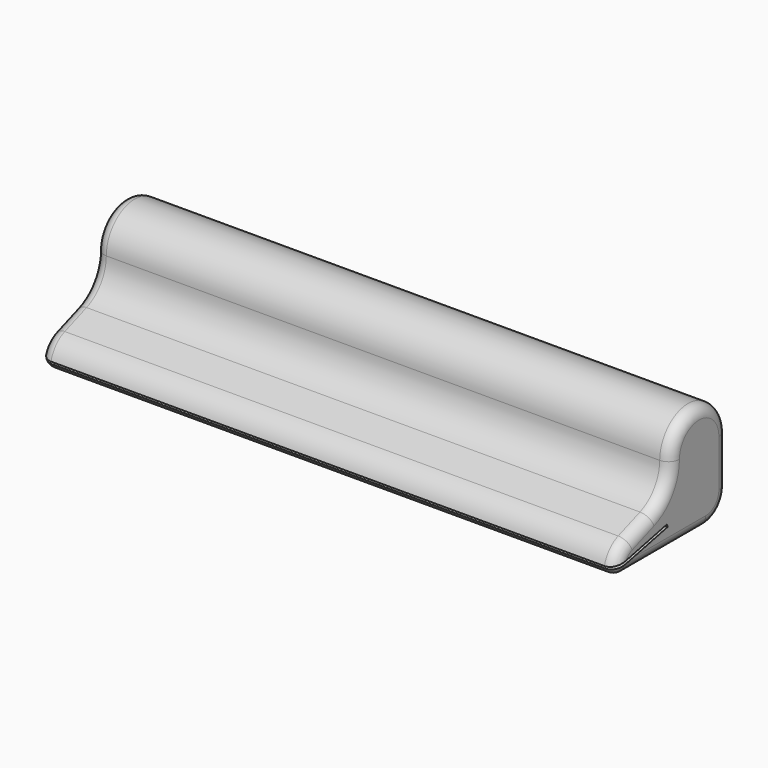
from build123d import *

# Parameters (mm, degrees)
F1_DEPTH     = 105
F2_T1_DEPTH  = 111.9389319908
F3_T1_DEPTH  = 130
F3_T3_DEPTH  = 125.8562768937
F4_T1_DEPTH  = 5.296560543
F4_T3_DEPTH  = 8.5
F4_T5_DEPTH  = 18.6122136018
F4_T8_ANGLE  = 69.7242191632
F4_T10_ANGLE = 180
F4_T12_ANGLE = 89.9999999974
F4_T16_ANGLE = 208.8901224768
F4_T19_ANGLE = 180
F4_T21_ANGLE = 89.9999999974
F4_T25_ANGLE = 208.8901224768
F4_T30_ANGLE = 113.8427963729
F4_T33_ANGLE = 69.7242191632
F4_T37_ANGLE = 113.8427963729


# Not quite as in the source:
# - a fillet or chamfer that OpenCascade refuses, or shapes differently, is made with other operations: its cross-section is extruded or revolved along the edge and cut away or added


with BuildPart() as f1:
    # F0 (on Right) → F1 (new body)
    with BuildSketch(Plane.YZ):
        with BuildLine():
            Line((13.561162162, 9.2741414115), (25, 13.5))
            ThreePointArc((25, 13.5), (18.5, 20), (12, 13.5))
            ThreePointArc((12, 13.5), (12.4027692373, 11.2474953881), (13.561162162, 9.2741414115))
        make_face()
        with BuildLine():
            ThreePointArc((13.561162162, 9.2741414115), (20.7525046119, 7.4027692373), (25, 13.5))
            Line((25, 13.5), (13.561162162, 9.2741414115))
        make_face()
        with BuildLine():
            Line((-0.4338704951, 1.1744297951), (0, 0))
            Line((0, 0), (25, 0))
            Line((25, 0), (25, 13.5))
            ThreePointArc((25, 13.5), (20.7525046119, 7.4027692373), (13.561162162, 9.2741414115))
            Line((13.561162162, 9.2741414115), (7.4949907763, 7.033111089))
            Line((7.4949907763, 7.033111089), (-1.3861566842, 3.7521420078))
            Line((-1.3861566842, 3.7521420078), (-0.6088429001, 1.6480568521))
            Line((-0.6088429001, 1.6480568521), (11.1854472535, 4.2144059557))
            Line((11.1854472535, 4.2144059557), (11.2917559365, 3.7258381877))
            Line((11.2917559365, 3.7258381877), (-0.4338704951, 1.1744297951))
        make_face()
        with BuildLine():
            Line((7.4949907763, 7.033111089), (13.561162162, 9.2741414115))
            ThreePointArc((13.561162162, 9.2741414115), (12.4027692373, 11.2474953881), (12, 13.5))
            ThreePointArc((12, 13.5), (10.7627204534, 9.559322384), (7.4949907763, 7.033111089))
        make_face()
    extrude(amount=F1_DEPTH)

    # F2: fillet of radius 2 on 1 edges, made by hand

    # F2_s2 → F2_t1 (cut)
    with BuildSketch(Plane.YZ.offset(-3.4694659954)):
        with BuildLine():
            ThreePointArc((-0.4338704951, 1.1744297951), (0.3040752765, 0.3190567514), (1.3877863982, 0))
            Line((1.3877863982, 0), (0, 0))
            Line((0, 0), (-0.4338704951, 1.1744297951))
        make_face()
    extrude(amount=F2_T1_DEPTH, mode=Mode.SUBTRACT)

    # F3: fillet of radius 5 on 2 edges, made by hand

    # F3_s2 → F3_t1 (cut)
    with BuildSketch(Plane.YZ.offset(-12.5)):
        with BuildLine():
            ThreePointArc((25, 5), (23.5355339059, 1.4644660941), (20, 0))
            Line((20, 0), (25, 0))
            Line((25, 0), (25, 5))
        make_face()
    extrude(amount=F3_T1_DEPTH, mode=Mode.SUBTRACT)

    # F3_s4 → F3_t3 (cut)
    with BuildSketch(Plane.YZ.offset(-10.4281384468)):
        with BuildLine():
            ThreePointArc((2.5266289487, 5.197645389), (0.5119597794, 3.8176424022), (-0.6088429001, 1.6480568521))
            Line((-0.6088429001, 1.6480568521), (-1.3861566842, 3.7521420078))
            Line((-1.3861566842, 3.7521420078), (2.5266289487, 5.197645389))
        make_face()
    extrude(amount=F3_T3_DEPTH, mode=Mode.SUBTRACT)

    # F4: fillet of radius 2 on 16 edges, made by hand

    # F4_s2 → F4_t1 (cut)
    with BuildSketch(Plane(origin=(0, 8.8811474605, 3.2809690812), x_dir=(1, 0, 0), z_dir=(0, -0.938035502, -0.3465391711))):
        with BuildLine():
            ThreePointArc((103, 4), (104.4142135624, 3.4142135624), (105, 2))
            Line((105, 2), (105.04, 2))
            Line((105.04, 2), (105.04, 4.04))
            Line((105.04, 4.04), (103, 4.04))
            Line((103, 4.04), (103, 4))
        make_face()
        with BuildLine():
            ThreePointArc((2, 4), (0.5857864376, 3.4142135624), (0, 2))
            Line((0, 2), (-0.04, 2))
            Line((-0.04, 2), (-0.04, 4.04))
            Line((-0.04, 4.04), (2, 4.04))
            Line((2, 4.04), (2, 4))
        make_face()
    extrude(amount=F4_T1_DEPTH, mode=Mode.SUBTRACT)

    # F4_s4 → F4_t3 (cut)
    with BuildSketch(Plane.XY.offset(5)):
        with BuildLine():
            ThreePointArc((105, 23), (104.4142135624, 24.4142135624), (103, 25))
            Line((103, 25), (103, 25.04))
            Line((103, 25.04), (105.04, 25.04))
            Line((105.04, 25.04), (105.04, 23))
            Line((105.04, 23), (105, 23))
        make_face()
        with BuildLine():
            ThreePointArc((0, 23), (0.5857864376, 24.4142135624), (2, 25))
            Line((2, 25), (2, 25.04))
            Line((2, 25.04), (-0.04, 25.04))
            Line((-0.04, 25.04), (-0.04, 23))
            Line((-0.04, 23), (0, 23))
        make_face()
    extrude(amount=F4_T3_DEPTH, mode=Mode.SUBTRACT)

    # F4_s6 → F4_t5 (cut)
    with BuildSketch(Plane.XZ.offset(-20)):
        with BuildLine():
            ThreePointArc((105, 2), (104.4142135624, 0.5857864376), (103, 0))
            Line((103, 0), (103, -0.04))
            Line((103, -0.04), (105.04, -0.04))
            Line((105.04, -0.04), (105.04, 2))
            Line((105.04, 2), (105, 2))
        make_face()
        with BuildLine():
            ThreePointArc((0, 2), (0.5857864376, 0.5857864376), (2, 0))
            Line((2, 0), (2, -0.04))
            Line((2, -0.04), (-0.04, -0.04))
            Line((-0.04, -0.04), (-0.04, 2))
            Line((-0.04, 2), (0, 2))
        make_face()
    extrude(amount=F4_T5_DEPTH, mode=Mode.SUBTRACT)

    # F4_s7 → F4_t8 (revolve, cut)
    with BuildSketch(Plane.XY.offset(13.5)):
        with BuildLine():
            ThreePointArc((105, 14), (104.4142135624, 12.5857864376), (103, 12))
            Line((103, 12), (103, 11.96))
            Line((103, 11.96), (105.04, 11.96))
            Line((105.04, 11.96), (105.04, 14))
            Line((105.04, 14), (105, 14))
        make_face()
    revolve(axis=Axis((105, 5.1059230727, 13.5), (-1, 0, 0)), revolution_arc=F4_T8_ANGLE, mode=Mode.SUBTRACT)

    # F4_s9 → F4_t10 (revolve, cut)
    with BuildSketch(Plane.XY.offset(13.5)):
        with BuildLine():
            ThreePointArc((105, 23), (104.4142135624, 24.4142135624), (103, 25))
            Line((103, 25), (103, 25.04))
            Line((103, 25.04), (105.04, 25.04))
            Line((105.04, 25.04), (105.04, 23))
            Line((105.04, 23), (105, 23))
        make_face()
    revolve(axis=Axis((105, 18.5, 13.5), (1, 0, 0)), revolution_arc=F4_T10_ANGLE, mode=Mode.SUBTRACT)

    # F4_s11 → F4_t12 (revolve, cut)
    with BuildSketch(Plane.XY.offset(5.0000000001)):
        with BuildLine():
            ThreePointArc((105, 23), (104.4142135624, 24.4142135624), (103, 25))
            Line((103, 25), (103, 25.04))
            Line((103, 25.04), (105.04, 25.04))
            Line((105.04, 25.04), (105.04, 23))
            Line((105.04, 23), (105, 23))
        make_face()
    revolve(axis=Axis((105, 19.9999999999, 5.0000000001), (-1, 0, 0)), revolution_arc=F4_T12_ANGLE, mode=Mode.SUBTRACT)


with BuildPart() as f4_tool14:
    # F4_s15 → F4_t16 (revolve)
    with BuildSketch(Plane.XZ.offset(-1.387786398)):
        with BuildLine():
            ThreePointArc((105, 2), (104.4142135624, 0.5857864376), (103, 0))
            Line((103, 0), (103, -0.04))
            Line((103, -0.04), (105.04, -0.04))
            Line((105.04, -0.04), (105.04, 2))
            Line((105.04, 2), (105, 2))
        make_face()
    revolve(axis=Axis((105, 1.387786398, 1.9999999997), (-1, 0, 0)), revolution_arc=F4_T16_ANGLE)

    split(bisect_by=Plane(origin=(0, -0.2636084299, 1.2114775439), x_dir=(1, 0, 0), z_dir=(0, 0.212617366, -0.977135536)), keep=Keep.TOP)


with BuildPart() as f1_1:
    add(f1.part)

    # F4_t13: cut F4_tool14
    add(f4_tool14.part, mode=Mode.SUBTRACT)

    # F4_s18 → F4_t19 (revolve, cut)
    with BuildSketch(Plane.XY.offset(13.5)):
        with BuildLine():
            ThreePointArc((0, 23), (0.5857864376, 24.4142135624), (2, 25))
            Line((2, 25), (2, 25.04))
            Line((2, 25.04), (-0.04, 25.04))
            Line((-0.04, 25.04), (-0.04, 23))
            Line((-0.04, 23), (0, 23))
        make_face()
    revolve(axis=Axis((0, 18.5, 13.5), (1, 0, 0)), revolution_arc=F4_T19_ANGLE, mode=Mode.SUBTRACT)

    # F4_s20 → F4_t21 (revolve, cut)
    with BuildSketch(Plane.XY.offset(5.0000000001)):
        with BuildLine():
            ThreePointArc((0, 23), (0.5857864376, 24.4142135624), (2, 25))
            Line((2, 25), (2, 25.04))
            Line((2, 25.04), (-0.04, 25.04))
            Line((-0.04, 25.04), (-0.04, 23))
            Line((-0.04, 23), (0, 23))
        make_face()
    revolve(axis=Axis((0, 19.9999999999, 5.0000000001), (-1, 0, 0)), revolution_arc=F4_T21_ANGLE, mode=Mode.SUBTRACT)


with BuildPart() as f4_tool23:
    # F4_s24 → F4_t25 (revolve)
    with BuildSketch(Plane.XZ.offset(-1.387786398)):
        with BuildLine():
            ThreePointArc((0, 2), (0.5857864376, 0.5857864376), (2, 0))
            Line((2, 0), (2, -0.04))
            Line((2, -0.04), (-0.04, -0.04))
            Line((-0.04, -0.04), (-0.04, 2))
            Line((-0.04, 2), (0, 2))
        make_face()
    revolve(axis=Axis((0, 1.387786398, 1.9999999997), (-1, 0, 0)), revolution_arc=F4_T25_ANGLE)

    split(bisect_by=Plane(origin=(0, -0.2636084299, 1.2114775439), x_dir=(1, 0, 0), z_dir=(0, 0.212617366, -0.977135536)), keep=Keep.TOP)


with BuildPart() as f1_2:
    add(f1_1.part)

    # F4_t22: cut F4_tool23
    add(f4_tool23.part, mode=Mode.SUBTRACT)


with BuildPart() as f4_tool28:
    # F4_s29 → F4_t30 (revolve)
    with BuildSketch(Plane(origin=(0, 1.8105345855, -1.8671150167), x_dir=(1, 0, 0), z_dir=(0, 0.6961456006, -0.7179006218))):
        with BuildLine():
            ThreePointArc((0, -0.4110434567), (0.5857864376, 1.0031701057), (2, 1.5889565433))
            Line((2, 1.5889565433), (2, 1.6289565433))
            Line((2, 1.6289565433), (-0.04, 1.6289565433))
            Line((-0.04, 1.6289565433), (-0.04, -0.4110434567))
            Line((-0.04, -0.4110434567), (0, -0.4110434567))
        make_face()
    revolve(axis=Axis((0, 4.259324804, 0.5074678792), (-1, 0, 0)), revolution_arc=F4_T30_ANGLE)

    split(bisect_by=Plane(origin=(0, -0.3699171129, 1.7000453119), x_dir=(1, 0, 0), z_dir=(0, -0.212617366, 0.977135536)), keep=Keep.TOP)


with BuildPart() as f1_3:
    add(f1_2.part)

    # F4_t27: cut F4_tool28
    add(f4_tool28.part, mode=Mode.SUBTRACT)

    # F4_s32 → F4_t33 (revolve, cut)
    with BuildSketch(Plane.XY.offset(13.5)):
        with BuildLine():
            ThreePointArc((0, 14), (0.5857864376, 12.5857864376), (2, 12))
            Line((2, 12), (2, 11.96))
            Line((2, 11.96), (-0.04, 11.96))
            Line((-0.04, 11.96), (-0.04, 14))
            Line((-0.04, 14), (0, 14))
        make_face()
    revolve(axis=Axis((0, 5.1059230727, 13.5), (-1, 0, 0)), revolution_arc=F4_T33_ANGLE, mode=Mode.SUBTRACT)


with BuildPart() as f4_tool35:
    # F4_s36 → F4_t37 (revolve)
    with BuildSketch(Plane(origin=(0, 1.8105345855, -1.8671150167), x_dir=(1, 0, 0), z_dir=(0, 0.6961456006, -0.7179006218))):
        with BuildLine():
            ThreePointArc((103, 1.5889565433), (104.4142135624, 1.0031701057), (105, -0.4110434567))
            Line((105, -0.4110434567), (105.04, -0.4110434567))
            Line((105.04, -0.4110434567), (105.04, 1.6289565433))
            Line((105.04, 1.6289565433), (103, 1.6289565433))
            Line((103, 1.6289565433), (103, 1.5889565433))
        make_face()
    revolve(axis=Axis((105, 4.259324804, 0.5074678792), (-1, 0, 0)), revolution_arc=F4_T37_ANGLE)

    split(bisect_by=Plane(origin=(0, -0.3699171129, 1.7000453119), x_dir=(1, 0, 0), z_dir=(0, -0.212617366, 0.977135536)), keep=Keep.TOP)


with BuildPart() as f1_4:
    add(f1_3.part)

    # F4_t34: cut F4_tool35
    add(f4_tool35.part, mode=Mode.SUBTRACT)


solid = f1_4.part
